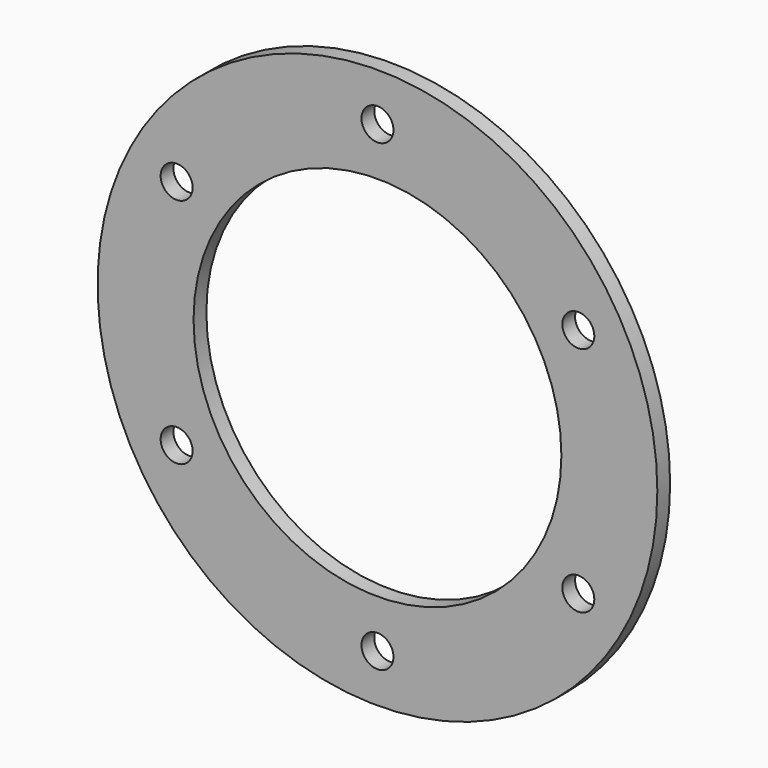
from build123d import *

# Parameters (mm, degrees)
F0_R            = 87.5
F0_R_2          = 57.5
F1_DEPTH        = 5
F2_R            = 5
F3_DEPTH        = 5.001
F3_COPIES_COUNT = 6


# Not quite as in the source:
# - a pattern or mirror of a feature is missing from the dataset's text; its kind, count and spacing are read off the source's solid


with BuildPart() as f1:
    # F0 (on Front) → F1 (new body)
    with BuildSketch(Plane.XZ):
        Circle(F0_R)
        Circle(F0_R_2, mode=Mode.SUBTRACT)
    extrude(amount=F1_DEPTH)

    # F2 (on face) → F3 (cut, through all)
    with BuildSketch(Plane.XZ.offset(5)):
        with Locations((0, 72.5)):
            Circle(F2_R)
    f3 = extrude(amount=-F3_DEPTH, mode=Mode.SUBTRACT)

    # F3_copies: F3 ×6 about axis
    f3_copies_axis = Axis((0, 0, 0), (0, 1, 0))
    for i in range(1, F3_COPIES_COUNT):
        add(f3.rotate(f3_copies_axis, i * 360 / F3_COPIES_COUNT), mode=Mode.SUBTRACT)


solid = f1.part
